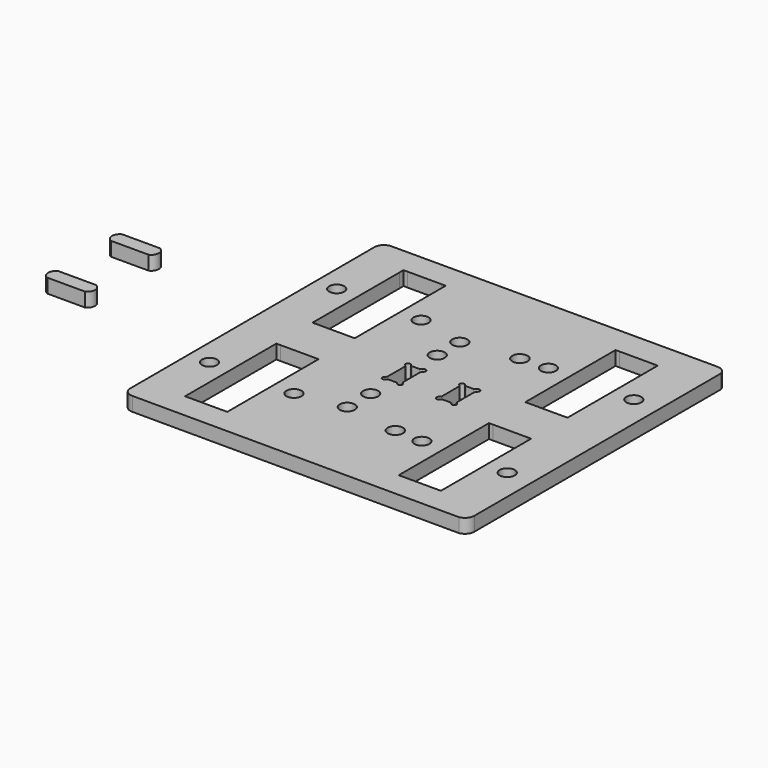
from build123d import *

# Parameters (mm, degrees)
F0_R     = 1.605
F0_R_2   = 1.606
F0_R_3   = 1.6345849858
F1_DEPTH = 3


# Not quite as in the source:
# - ends of sketch curves that miss each other by under 0.0002 mm in the source are joined


with BuildPart() as f1:
    # F0 (on Top) → F1 (new body)
    with BuildSketch(Plane.XY):
        with BuildLine():
            Line((-16.9731467252, 71.6227536132), (-16.9016096355, 6.3827649274))
            ThreePointArc((-16.9016096355, 6.3827649274), (-16.3498938581, 4.9693411595), (-14.9364701023, 4.4176253513))
            Line((-14.9364701023, 4.4176253513), (54.9699635075, 4.2401110439))
            ThreePointArc((54.9699635075, 4.2401110439), (56.1908043606, 4.9140051596), (56.6761346812, 6.2213077824))
            Line((56.6761346812, 6.2213077824), (56.6761346812, 71.9221415992))
            ThreePointArc((56.6761346812, 71.9221415992), (56.0022405655, 73.1429824523), (54.6949379427, 73.6283127729))
            Line((54.6949379427, 73.6283127729), (-14.9697846716, 73.6283133561))
            ThreePointArc((-14.9697846716, 73.6283133561), (-16.3871527066, 73.0407650431), (-16.9731467252, 71.6227536132))
        make_face()
        with Locations((-12.4550571863, 21.9445816246)):
            Circle(F0_R, mode=Mode.SUBTRACT)
        Polygon((-7.9783601332, 34.1825555709), (-7.115187118, 34.1825555379), (0.1649951569, 34.1825525659), (1.0367866374, 34.182552206), (1.0367866374, 33.0762614296), (1.0367866374, 10.6706960983), (1.0367836324, 9.8032168566), (0.1693013857, 9.8032168566), (-7.1108808916, 9.8032138516), (-7.9783601332, 9.8032168566), (-7.9783601332, 10.6706981016), (-7.9783601332, 33.0762594262), align=None, mode=Mode.SUBTRACT)
        with Locations((5.5752103113, 21.9445816246)):
            Circle(F0_R, mode=Mode.SUBTRACT)
        with Locations((15.5920255878, 23.6635602825)):
            Circle(F0_R_2, mode=Mode.SUBTRACT)
        with Locations((27.1354746317, 22.0575592808)):
            Circle(F0_R_3, mode=Mode.SUBTRACT)
        with Locations((15.5920255878, 29.8969212558)):
            Circle(F0_R_2, mode=Mode.SUBTRACT)
        with BuildLine():
            Line((13.9392921361, 36.5909245116), (13.9392921361, 41.066387493))
            ThreePointArc((13.9392921361, 41.066387493), (13.8721927186, 41.3168069715), (13.6888735611, 41.5001272745))
            ThreePointArc((13.6888735611, 41.5001272745), (13.5851479016, 42.2880162976), (14.3730360405, 42.1842879889))
            ThreePointArc((14.3730360405, 42.1842879889), (14.5563571581, 42.0009675875), (14.8067773878, 41.9338677363))
            Line((14.8067773878, 41.9338677363), (16.3772807995, 41.9338707414))
            ThreePointArc((16.3772807995, 41.9338707414), (16.6277006536, 42.0009703757), (16.8110210147, 42.1842900676))
            ThreePointArc((16.8110210147, 42.1842900676), (17.5989095566, 42.2880150233), (17.4951817292, 41.5001270874))
            ThreePointArc((17.4951817292, 41.5001270874), (17.3118610192, 41.3168059362), (17.2447610428, 41.0663854897))
            Line((17.2447610428, 41.0663854897), (17.2447640478, 36.5909235099))
            ThreePointArc((17.2447640478, 36.5909235099), (17.311863557, 36.3405038727), (17.4951829403, 36.1571835451))
            ThreePointArc((17.4951829403, 36.1571835451), (17.5989083298, 35.3692947528), (16.8110203938, 35.4730225802))
            ThreePointArc((16.8110203938, 35.4730225802), (16.6276992427, 35.6563432902), (16.3772787961, 35.7234432666))
            Line((16.3772787961, 35.7234432666), (14.8067723794, 35.7234402616))
            ThreePointArc((14.8067723794, 35.7234402616), (14.556352901, 35.6563408441), (14.3730325979, 35.4730216866))
            ThreePointArc((14.3730325979, 35.4730216866), (13.5851437519, 35.36929585), (13.6888718835, 36.157184166))
            ThreePointArc((13.6888718835, 36.157184166), (13.8721922849, 36.3405042819), (13.9392921361, 36.5909245116))
        make_face(mode=Mode.SUBTRACT)
        with BuildLine():
            Line((25.4827411801, 36.5909245116), (25.4827411801, 41.066387493))
            ThreePointArc((25.4827411801, 41.066387493), (25.4156417626, 41.3168069715), (25.2323226051, 41.5001272745))
            ThreePointArc((25.2323226051, 41.5001272745), (25.1285969456, 42.2880162976), (25.9164850845, 42.1842879889))
            ThreePointArc((25.9164850845, 42.1842879889), (26.0998059852, 42.0009677127), (26.3502264318, 41.9338677363))
            Line((26.3502264318, 41.9338677363), (27.9207298435, 41.9338707414))
            ThreePointArc((27.9207298435, 41.9338707414), (28.1711496975, 42.0009703757), (28.3544700587, 42.1842900676))
            ThreePointArc((28.3544700587, 42.1842900676), (29.1423586006, 42.2880150233), (29.0386307731, 41.5001270874))
            ThreePointArc((29.0386307731, 41.5001270874), (28.8553100632, 41.3168059362), (28.7882100868, 41.0663854897))
            Line((28.7882100868, 41.0663854897), (28.7882130918, 36.5909235099))
            ThreePointArc((28.7882130918, 36.5909235099), (28.855312601, 36.3405038727), (29.0386319843, 36.1571835451))
            ThreePointArc((29.0386319843, 36.1571835451), (29.1423571967, 35.3692945757), (28.3544691874, 35.473023014))
            ThreePointArc((28.3544691874, 35.473023014), (28.1711482867, 35.6563432902), (27.9207278401, 35.7234432666))
            Line((27.9207278401, 35.7234432666), (26.3502214234, 35.7234402616))
            ThreePointArc((26.3502214234, 35.7234402616), (26.0998019449, 35.6563408441), (25.9164816419, 35.4730216866))
            ThreePointArc((25.9164816419, 35.4730216866), (25.1285927959, 35.36929585), (25.2323209275, 36.157184166))
            ThreePointArc((25.2323209275, 36.157184166), (25.4156413288, 36.3405042819), (25.4827411801, 36.5909245116))
        make_face(mode=Mode.SUBTRACT)
        with Locations((33.0016662521, 21.8139863938)):
            Circle(F0_R, mode=Mode.SUBTRACT)
        Polygon((37.6654533742, 33.9035358044), (38.5227925937, 33.9035361797), (45.8029748711, 33.9035331747), (46.6806001449, 33.9035361797), (46.6806001449, 33.0762614296), (46.6806001449, 10.6706960983), (46.6805971399, 9.8032168566), (45.8131148932, 9.8032168566), (38.5329326158, 9.8032138516), (37.6654533742, 9.8032168566), (37.6654533742, 10.6706981016), (37.6654533742, 33.0762594262), align=None, mode=Mode.SUBTRACT)
        with Locations((51.2396564549, 21.8139863938)):
            Circle(F0_R, mode=Mode.SUBTRACT)
        with Locations((-12.4550571863, 55.8864670325)):
            Circle(F0_R, mode=Mode.SUBTRACT)
        Polygon((-7.1122992726, 68.1489150636), (0.1678830047, 68.1489180686), (1.0252222242, 68.1489150636), (1.0252222242, 67.1334313662), (1.0252222242, 44.7278700416), (1.0252222242, 43.8603887966), (0.1577429826, 43.8603857915), (-7.1224392948, 43.8603887966), (-7.9899215414, 43.8603887966), (-7.9899245465, 44.7278680382), (-7.9899245465, 67.1334333695), (-7.9899215414, 68.1489154258), align=None, mode=Mode.SUBTRACT)
        with Locations((5.5752103113, 55.8864670325)):
            Circle(F0_R, mode=Mode.SUBTRACT)
        with Locations((15.5920255878, 47.6820342113)):
            Circle(F0_R_2, mode=Mode.SUBTRACT)
        with Locations((15.5920255878, 53.7140061118)):
            Circle(F0_R_2, mode=Mode.SUBTRACT)
        with Locations((27.1354786385, 55.3315615099)):
            Circle(F0_R_3, mode=Mode.SUBTRACT)
        with Locations((33.0016662521, 55.6207377599)):
            Circle(F0_R, mode=Mode.SUBTRACT)
        Polygon((37.6654533742, 67.7102878997), (38.5227925937, 67.7102875459), (45.8029748711, 67.7102845408), (46.6806001449, 67.7102875459), (46.6806001449, 66.8830127957), (46.6806001449, 44.4774474644), (46.6805971399, 43.6099682228), (45.8131148932, 43.6099682228), (38.5329326158, 43.6099652177), (37.6654533742, 43.6099682228), (37.6654533742, 44.4774494677), (37.6654533742, 66.8830107923), align=None, mode=Mode.SUBTRACT)
        with Locations((51.2396564549, 55.6207377599)):
            Circle(F0_R, mode=Mode.SUBTRACT)
    extrude(amount=F1_DEPTH)


with BuildPart() as f1b:
    # F0 (on Top) → F1, piece 2 (new body)
    with BuildSketch(Plane.XY):
        with BuildLine():
            ThreePointArc((-44.6885697404, 45.9386355595), (-43.6868882127, 47.441157851), (-44.6885697404, 48.9436801425))
            Line((-44.6885697404, 48.9436801425), (-52.7020219615, 48.9436801425))
            ThreePointArc((-52.7020219615, 48.9436801425), (-53.7037034892, 47.441157851), (-52.7020219615, 45.9386355595))
            Line((-52.7020219615, 45.9386355595), (-44.6885697404, 45.9386355595))
        make_face()
    extrude(amount=F1_DEPTH)


with BuildPart() as f1c:
    # F0 (on Top) → F1, piece 3 (new body)
    with BuildSketch(Plane.XY):
        with BuildLine():
            ThreePointArc((-44.6885697404, 28.9100495895), (-43.6868882127, 30.412571881), (-44.6885697404, 31.9150941725))
            Line((-44.6885697404, 31.9150941725), (-52.7020219615, 31.9150941725))
            ThreePointArc((-52.7020219615, 31.9150941725), (-53.7037034892, 30.412571881), (-52.7020219615, 28.9100495895))
            Line((-52.7020219615, 28.9100495895), (-44.6885697404, 28.9100495895))
        make_face()
    extrude(amount=F1_DEPTH)


solid = Compound([f1.part, f1b.part, f1c.part])
